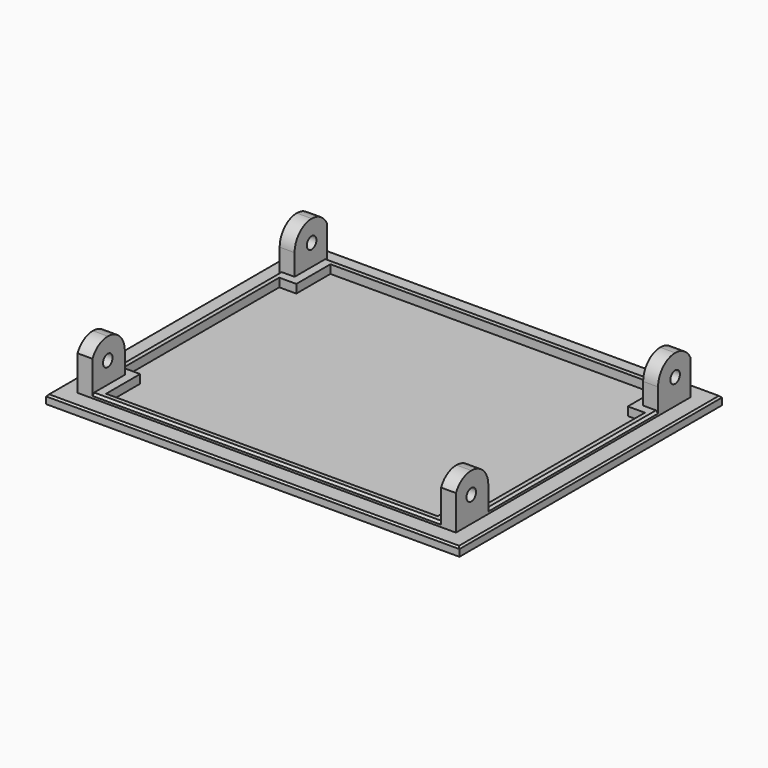
from build123d import *

# Parameters (mm, degrees)
F0_W      = 97
F0_H      = 77
F1_DEPTH  = 2
F2_W      = 89.8
F2_H      = 69.8
F3_DEPTH  = 1
F4_W      = 4
F4_H      = 10
F5_DEPTH  = 10
F6_R      = 4.99999
F7_R      = 1.4
F8_DEPTH  = 93.401
F10_DEPTH = 2
F11_W     = 97
F11_H     = 77
F11_W_2   = 88.8
F11_H_2   = 68.8
F12_DEPTH = 11.001
F13_SIZE  = 0.5
F14_SIZE  = 0.4


# Not quite as in the source:
# - a fillet or chamfer is up to 0.001 mm smaller than in the source, because OpenCascade refuses the exact size


with BuildPart() as f1:
    # F0 (on Top) → F1 (new body)
    with BuildSketch(Plane.XY):
        Rectangle(F0_W, F0_H)
    extrude(amount=F1_DEPTH)

    # F2 (on face) → F3 (join)
    with BuildSketch(Plane.XY.offset(2)):
        Rectangle(F2_W, F2_H)
    extrude(amount=F3_DEPTH)

    # F4 (on face) → F5 (join)
    with BuildSketch(Plane.XY.offset(3)):
        with Locations((-42.9, 29.9)):
            Rectangle(F4_W, F4_H)
        with Locations((42.9, 29.9)):
            Rectangle(F4_W, F4_H)
        with Locations((-42.9, -29.9)):
            Rectangle(F4_W, F4_H)
        with Locations((42.9, -29.9)):
            Rectangle(F4_W, F4_H)
    extrude(amount=F5_DEPTH)

    # F6 (radius 5 in the source; OpenCascade refuses exactly that, so slightly less here)
    f6_edges = [f1.edges().sort_by_distance(p)[0] for p in [
        (42.9, 34.9, 13),
        (42.9, 24.9, 13),
        (42.9, -24.9, 13),
        (42.9, -34.9, 13),
        (-42.9, -24.9, 13),
        (-42.9, -34.9, 13),
        (-42.9, 34.9, 13),
        (-42.9, 24.9, 13),
    ]]
    fillet(f6_edges, radius=F6_R)

    # F7 (on face) → F8 (cut, through all)
    with BuildSketch(Plane(origin=(-44.9, 0, 0), x_dir=(0, -1, 0), z_dir=(-1, 0, 0))):
        with Locations((-29.9, 8)):
            Circle(F7_R)
        with Locations((29.9, 8)):
            Circle(F7_R)
    extrude(amount=-F8_DEPTH, mode=Mode.SUBTRACT)

    # F9 (on face) → F10 (cut)
    with BuildSketch(Plane.XY.offset(3)):
        Polygon((-42.9, -22.9), (-38.9, -22.9), (-38.9, -32.9), (38.9, -32.9), (38.9, -22.9), (42.9, -22.9), (42.9, 22.9), (38.9, 22.9), (38.9, 32.9), (-38.9, 32.9), (-38.9, 22.9), (-42.9, 22.9), align=None)
    extrude(amount=-F10_DEPTH, mode=Mode.SUBTRACT)

    # F11 (on face) → F12 (cut, through all)
    with BuildSketch(Plane.XY.offset(2)):
        Rectangle(F11_W, F11_H)
        Rectangle(F11_W_2, F11_H_2, mode=Mode.SUBTRACT)
    extrude(amount=F12_DEPTH, mode=Mode.SUBTRACT)

    # F13
    f13_edges = [f1.edges().sort_by_distance(p)[0] for p in [
        (44.4, 0, 3),
        (0, -34.4, 3),
        (-44.4, 0, 3),
        (0, 34.4, 3),
    ]]
    chamfer(f13_edges, length=F13_SIZE)

    # F14
    f14_edges = [f1.edges().sort_by_distance(p)[0] for p in [
        (-48.5, 0, 2),
        (0, 38.5, 2),
        (48.5, 0, 2),
        (0, -38.5, 2),
    ]]
    chamfer(f14_edges, length=F14_SIZE)


solid = f1.part
